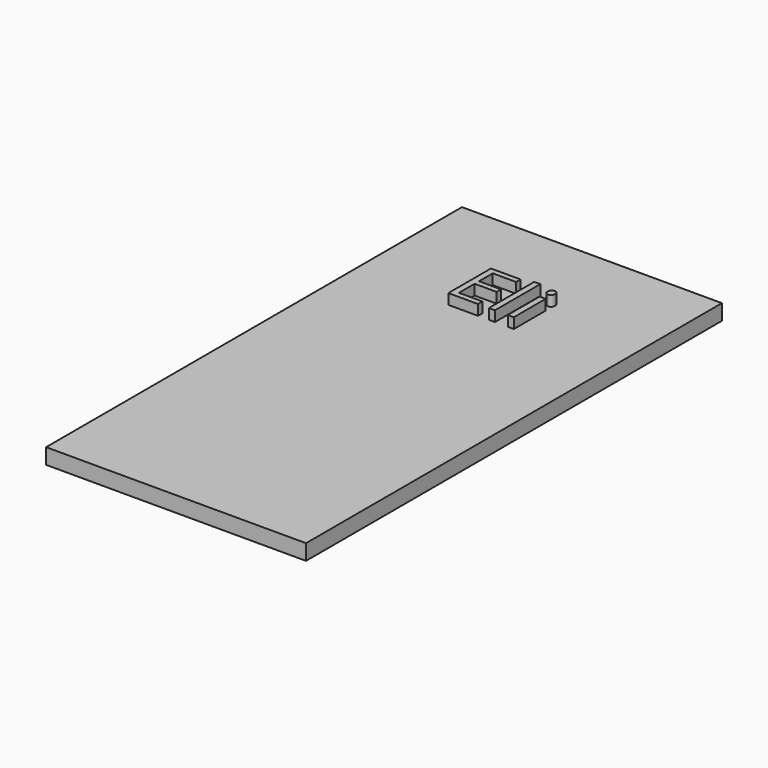
from build123d import *

# Parameters (mm, degrees)
F0_W         = 50
F0_H         = 100
F1_DEPTH     = 3
F2_TEXT_SIZE = 14.3402799343
F3_DEPTH     = 2


# Not quite as in the source:
# - Text() gives the source's letters only with a copy of the font that has no kerning and outlines rounded to 1/6400 em; it was checked with that copy


with BuildPart() as f1:
    # F0 (on Top) → F1 (new body)
    with BuildSketch(Plane.XY):
        Rectangle(F0_W, F0_H)
    extrude(amount=F1_DEPTH)

    # F2 (on face) → F3 (join)
    with BuildSketch(Plane.XY.offset(3)):
        with Locations((-8.1374985166, 23.8875020295)):
            Text('Eli', F2_TEXT_SIZE, font='Open Sans', text_align=(TextAlign.LEFT, TextAlign.BOTTOM))
    extrude(amount=F3_DEPTH)


solid = f1.part
